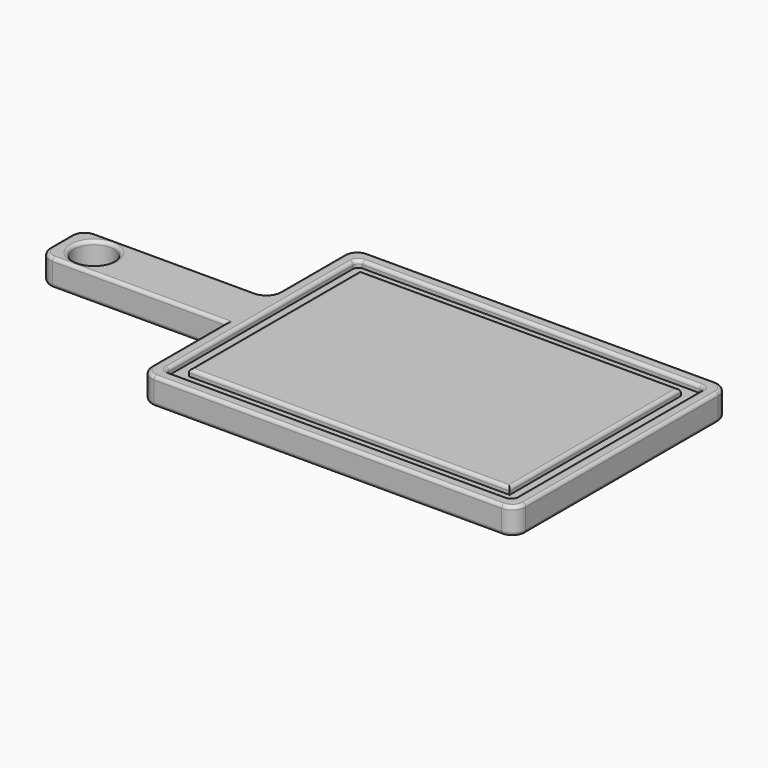
from build123d import *

# Parameters (mm, degrees)
F0_W     = 177.8
F0_H     = 50.8
F1_DEPTH = 25.4
F2_R     = 19.05
F3_DEPTH = 25.4
F5_DEPTH = 6.35
F6_R     = 5.08
F7_R     = 12.7
F8_R     = 3.17499


# Not quite as in the source:
# - a fillet or chamfer is up to 0.001 mm smaller than in the source, because OpenCascade refuses the exact size


with BuildPart() as f1:
    # F0 (on Top) → F1 (new body)
    with BuildSketch(Plane.XY):
        Polygon((0, 101.6), (0, 0), (355.6, 0), (355.6, 254), (0, 254), (0, 152.4), align=None)
        with Locations((-88.9, 127)):
            Rectangle(F0_W, F0_H)
    extrude(amount=F1_DEPTH)

    # F2 (on face) → F3 (cut)
    with BuildSketch(Plane.XY.offset(25.4)):
        with Locations((-146.05, 127)):
            Circle(F2_R)
    extrude(amount=-F3_DEPTH, mode=Mode.SUBTRACT)

    # F4 (on face) → F5 (cut)
    with BuildSketch(Plane.XY.offset(25.4)):
        Polygon((12.7, 101.6), (12.7, 12.7), (342.9, 12.7), (342.9, 241.3), (12.7, 241.3), (12.7, 152.4), align=None)
        Polygon((25.4, 101.6), (25.4, 152.4), (25.4, 228.6), (330.2, 228.6), (330.2, 25.4), (25.4, 25.4), align=None, mode=Mode.SUBTRACT)
    extrude(amount=-F5_DEPTH, mode=Mode.SUBTRACT)

    # F6
    f6_edges = [f1.edges().sort_by_distance(p)[0] for p in [
        (12.7, 241.3, 22.225),
        (342.9, 241.3, 22.225),
        (12.7, 12.7, 22.225),
        (342.9, 12.7, 22.225),
    ]]
    fillet(f6_edges, radius=F6_R)

    # F7
    f7_edges = [f1.edges().sort_by_distance(p)[0] for p in [
        (355.6, 0, 12.7),
        (0, 0, 12.7),
        (-177.8, 101.6, 12.7),
        (-177.8, 152.4, 12.7),
        (0, 152.4, 12.7),
        (0, 254, 12.7),
        (355.6, 254, 12.7),
    ]]
    fillet(f7_edges, radius=F7_R)

    # F8 (radius 3.175 in the source; OpenCascade refuses exactly that, so slightly less here)
    f8_edges = [f1.edges().sort_by_distance(p)[0] for p in [
        (177.8, 228.6, 25.4),
        (330.2, 127, 25.4),
        (177.8, 25.4, 25.4),
        (25.4, 127, 25.4),
        (0, 57.15, 25.4),
        (3.719744, 3.719744, 25.4),
        (-82.55, 101.6, 25.4),
        (177.8, 0, 25.4),
        (-174.080256, 105.319744, 25.4),
        (351.880256, 3.719744, 25.4),
        (-177.8, 127, 25.4),
        (355.6, 127, 25.4),
        (-174.080256, 148.680256, 25.4),
        (351.880256, 250.280256, 25.4),
        (-88.9, 152.4, 25.4),
        (177.8, 254, 25.4),
        (-3.719744, 156.119744, 25.4),
        (3.719744, 250.280256, 25.4),
        (0, 203.2, 25.4),
        (177.8, 12.7, 25.4),
        (14.187898, 14.187898, 25.4),
        (341.412102, 14.187898, 25.4),
        (12.7, 127, 25.4),
        (342.9, 127, 25.4),
        (14.187898, 239.812102, 25.4),
        (341.412102, 239.812102, 25.4),
        (177.8, 241.3, 25.4),
        (-165.1, 127, 25.4),
        (0, 57.15, 0),
        (3.719744, 3.719744, 0),
        (-82.55, 101.6, 0),
        (177.8, 0, 0),
        (-174.080256, 105.319744, 0),
        (351.880256, 3.719744, 0),
        (-177.8, 127, 0),
        (355.6, 127, 0),
        (-174.080256, 148.680256, 0),
        (351.880256, 250.280256, 0),
        (-88.9, 152.4, 0),
        (177.8, 254, 0),
        (-3.719744, 156.119744, 0),
        (3.719744, 250.280256, 0),
        (0, 203.2, 0),
        (-165.1, 127, 0),
    ]]
    fillet(f8_edges, radius=F8_R)


solid = f1.part
